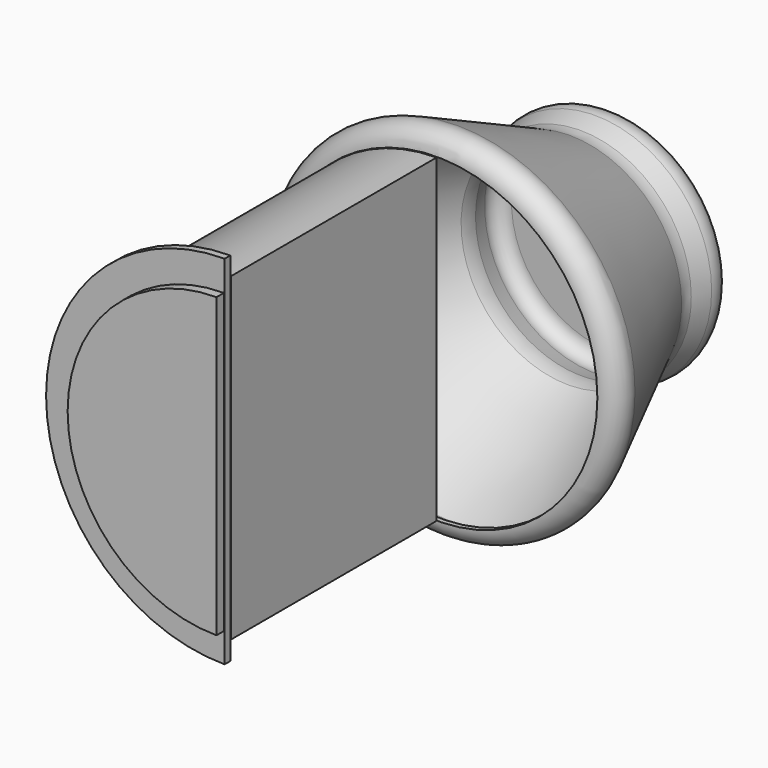
from build123d import *

# Parameters (mm, degrees)
F0_R          = 55.4946398795
F1_DEPTH      = 88
F1_TAPER      = -25
F1_DEPTH_BACK = 25
F1_TAPER_BACK = -17
F2_R          = 9.3955575751
F5_DEPTH      = 131
F6_T          = -2.5
F7_T          = -2.5
F10_DEPTH     = 3.6
F13_DEPTH     = 4.7


# Not quite as in the source:
# - a shell that OpenCascade refuses in one call is made with other operations: the cavity is built on its own and cut out


with BuildPart() as f1:
    # F0 (on Front) → F1 (new body, two sides)
    with BuildSketch(Plane.XZ) as f1_sk:
        Circle(F0_R)
    extrude(amount=F1_DEPTH, taper=F1_TAPER)
    extrude(f1_sk.sketch, amount=-F1_DEPTH_BACK, taper=F1_TAPER_BACK)

    # F2
    f2_edges = [f1.edges().sort_by_distance(p)[0] for p in [
        (-96.529714, -88, 0),
        (-63.137907, 25, 0),
        (-55.49464, 0, 0),
    ]]
    fillet(f2_edges, radius=F2_R)

    # F6: a shell. OpenCascade refuses it in one call, so the cavity is built on its own and cut out:
    # the body offset inwards by the wall thickness, plus a prism from it out through each open face.
    f6_core = offset(f1.part, amount=F6_T, mode=Mode.PRIVATE)
    f6_exits = [f6_core.faces().sort_by_distance(p)[0] for p in [
        (0, -85.5, 0),
    ]]
    add(f6_core, mode=Mode.SUBTRACT)
    extrude(f6_exits, amount=-F6_T, mode=Mode.SUBTRACT)


with BuildPart() as f5:
    # F4 (on offset) → F5 (new body)
    with BuildSketch(Plane.XZ.offset(88.4)):
        with BuildLine():
            Line((0, -81.64971785), (0, 81.64971785))
            ThreePointArc((0, 81.64971785), (-81.64971785, 0), (0, -81.64971785))
        make_face()
    extrude(amount=F5_DEPTH)

    # F7
    f7_openings = [f5.faces().sort_by_distance(p)[0] for p in [
        (-34.653217, -219.4, 0),
    ]]
    offset(amount=F7_T, openings=f7_openings)


with BuildPart() as f10:
    # F9 (on offset) → F10 (new body)
    with BuildSketch(Plane.XZ.offset(220)):
        with BuildLine():
            Line((0, -91.1385615924), (0, 91.1385615924))
            ThreePointArc((0, 91.1385615924), (-91.1385615924, 0), (0, -91.1385615924))
        make_face()
    extrude(amount=F10_DEPTH)


with BuildPart() as f13:
    # F12 (on offset) → F13 (new body)
    with BuildSketch(Plane.XZ.offset(224.1)):
        with BuildLine():
            Line((0, -75.9726215886), (0, 75.9726215886))
            ThreePointArc((0, 75.9726215886), (-75.9726215886, 0), (0, -75.9726215886))
        make_face()
    extrude(amount=F13_DEPTH)


solid = Compound([f1.part, f5.part, f10.part, f13.part])
